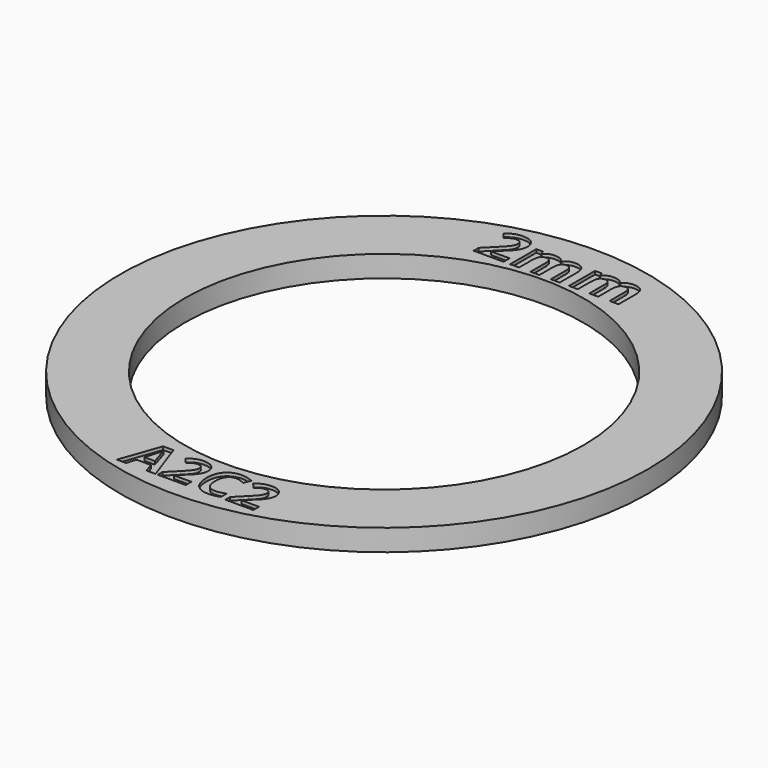
from build123d import *

# Parameters (mm, degrees)
F0_R           = 24.5
F0_R_2         = 18.5
F0_TEXT_SIZE   = 5.1974965673
F0_TEXT_SIZE_2 = 5.5555555556
F1_DEPTH       = 2
F2_DEPTH       = 0.3


# Not quite as in the source:
# - Text() gives the source's letters only with a copy of the font that has no kerning and outlines rounded to 1/6400 em; it was checked with that copy


with BuildPart() as f1:
    # F0 (on Top) → F1 (new body)
    with BuildSketch(Plane.XY):
        Circle(F0_R)
        Polygon((-2.9154707307, -22.8730905801), (-3.7633123583, -22.8730905801), (-4.0321203839, -21.9895161637), (-5.3850937091, -21.9895161637), (-5.6539017347, -22.8730905801), (-6.5017433622, -22.8730905801), (-5.1918118055, -19.1471352284), (-4.2302749405, -19.1471352284), align=None, mode=Mode.SUBTRACT)
        with BuildLine():
            Line((-0.1136952374, -22.2128460943), (-0.1136952374, -22.8730905801))
            Line((-0.1136952374, -22.8730905801), (-2.707570868, -22.8730905801))
            Line((-2.707570868, -22.8730905801), (-2.707570868, -22.3273534405))
            Line((-2.707570868, -22.3273534405), (-1.7760820301, -21.3861192965))
            add(Edge.make_bspline(
                [(-1.7760820301, -21.3861192965), (-1.3619065224, -20.9621984828), (-1.2352175436, -20.7985585518)],
                knots=[0, 0, 0, 1, 1, 1], degree=2))
            add(Edge.make_bspline(
                [(-1.2352175436, -20.7985585518), (-1.1085285648, -20.6349186208), (-1.0524930549, -20.4952359005)],
                knots=[0, 0, 0, 1, 1, 1], degree=2))
            add(Edge.make_bspline(
                [(-1.0524930549, -20.4952359005), (-0.996457545, -20.3555531803), (-0.996457545, -20.206125154)],
                knots=[0, 0, 0, 1, 1, 1], degree=2))
            add(Edge.make_bspline(
                [(-0.996457545, -20.206125154), (-0.996457545, -19.9827952234), (-1.1198980885, -19.8735665846)],
                knots=[0, 0, 0, 1, 1, 1], degree=2))
            add(Edge.make_bspline(
                [(-1.1198980885, -19.8735665846), (-1.243338632, -19.7643379458), (-1.4488021681, -19.7643379458)],
                knots=[0, 0, 0, 1, 1, 1], degree=2))
            add(Edge.make_bspline(
                [(-1.4488021681, -19.7643379458), (-1.6640110104, -19.7643379458), (-1.86703822, -19.8634152241)],
                knots=[0, 0, 0, 1, 1, 1], degree=2))
            add(Edge.make_bspline(
                [(-1.86703822, -19.8634152241), (-2.0700654297, -19.9624925024), (-2.2909590338, -20.1452169911)],
                knots=[0, 0, 0, 1, 1, 1], degree=2))
            Line((-2.2909590338, -20.1452169911), (-2.7173161741, -19.6400852935))
            add(Edge.make_bspline(
                [(-2.7173161741, -19.6400852935), (-2.4436354955, -19.4061979479), (-2.2633473333, -19.3099630505)],
                knots=[0, 0, 0, 1, 1, 1], degree=2))
            add(Edge.make_bspline(
                [(-2.2633473333, -19.3099630505), (-2.0830591711, -19.2137281532), (-1.869880601, -19.1617531875)],
                knots=[0, 0, 0, 1, 1, 1], degree=2))
            add(Edge.make_bspline(
                [(-1.869880601, -19.1617531875), (-1.6567020308, -19.1097782218), (-1.3927666583, -19.1097782218)],
                knots=[0, 0, 0, 1, 1, 1], degree=2))
            add(Edge.make_bspline(
                [(-1.3927666583, -19.1097782218), (-1.0451840753, -19.1097782218), (-0.7788123763, -19.2364672006)],
                knots=[0, 0, 0, 1, 1, 1], degree=2))
            add(Edge.make_bspline(
                [(-0.7788123763, -19.2364672006), (-0.5124406772, -19.3631561795), (-0.365042923, -19.5917648176)],
                knots=[0, 0, 0, 1, 1, 1], degree=2))
            add(Edge.make_bspline(
                [(-0.365042923, -19.5917648176), (-0.2176451688, -19.8203734556), (-0.2176451688, -20.1143568552)],
                knots=[0, 0, 0, 1, 1, 1], degree=2))
            add(Edge.make_bspline(
                [(-0.2176451688, -20.1143568552), (-0.2176451688, -20.3709832482), (-0.3077892498, -20.5955313421)],
                knots=[0, 0, 0, 1, 1, 1], degree=2))
            add(Edge.make_bspline(
                [(-0.3077892498, -20.5955313421), (-0.3979333309, -20.820079436), (-0.5871546903, -21.0559970536)],
                knots=[0, 0, 0, 1, 1, 1], degree=2))
            add(Edge.make_bspline(
                [(-0.5871546903, -21.0559970536), (-0.7763760497, -21.2919146713), (-1.253083938, -21.7288292265)],
                knots=[0, 0, 0, 1, 1, 1], degree=2))
            Line((-1.253083938, -21.7288292265), (-1.7306039352, -22.1779254142))
            Line((-1.7306039352, -22.1779254142), (-1.7306039352, -22.2128460943))
            Line((-1.7306039352, -22.2128460943), (-0.1136952374, -22.2128460943))
        make_face(mode=Mode.SUBTRACT)
        Circle(F0_R_2, mode=Mode.SUBTRACT)
        with BuildLine():
            add(Edge.make_bspline(
                [(2.5077920937, -19.8378337957), (2.2974559045, -19.7643379458), (2.0944286949, -19.7643379458)],
                knots=[0, 0, 0, 1, 1, 1], degree=2))
            add(Edge.make_bspline(
                [(2.0944286949, -19.7643379458), (1.6502051601, -19.7643379458), (1.4065725085, -20.0981146785)],
                knots=[0, 0, 0, 1, 1, 1], degree=2))
            add(Edge.make_bspline(
                [(1.4065725085, -20.0981146785), (1.1629398569, -20.4318914111), (1.1629398569, -21.0279792987)],
                knots=[0, 0, 0, 1, 1, 1], degree=2))
            add(Edge.make_bspline(
                [(1.1629398569, -21.0279792987), (1.1629398569, -22.2688816042), (2.0944286949, -22.2688816042)],
                knots=[0, 0, 0, 1, 1, 1], degree=2))
            add(Edge.make_bspline(
                [(2.0944286949, -22.2688816042), (2.4850530463, -22.2688816042), (3.0405354919, -22.0739754829)],
                knots=[0, 0, 0, 1, 1, 1], degree=2))
            Line((3.0405354919, -22.0739754829), (3.0405354919, -22.7334078599))
            add(Edge.make_bspline(
                [(3.0405354919, -22.7334078599), (2.5841303246, -22.9242534369), (2.0205267906, -22.9242534369)],
                knots=[0, 0, 0, 1, 1, 1], degree=2))
            add(Edge.make_bspline(
                [(2.0205267906, -22.9242534369), (1.2108542784, -22.9242534369), (0.7820608116, -22.4329275896)],
                knots=[0, 0, 0, 1, 1, 1], degree=2))
            add(Edge.make_bspline(
                [(0.7820608116, -22.4329275896), (0.3532673448, -21.9416017422), (0.3532673448, -21.0231066457)],
                knots=[0, 0, 0, 1, 1, 1], degree=2))
            add(Edge.make_bspline(
                [(0.3532673448, -21.0231066457), (0.3532673448, -20.4440730437), (0.5640095884, -20.0087827062)],
                knots=[0, 0, 0, 1, 1, 1], degree=2))
            add(Edge.make_bspline(
                [(0.5640095884, -20.0087827062), (0.7747518321, -19.5734923687), (1.1694367277, -19.3416352953)],
                knots=[0, 0, 0, 1, 1, 1], degree=2))
            add(Edge.make_bspline(
                [(1.1694367277, -19.3416352953), (1.5641216232, -19.1097782218), (2.0944286949, -19.1097782218)],
                knots=[0, 0, 0, 1, 1, 1], degree=2))
            add(Edge.make_bspline(
                [(2.0944286949, -19.1097782218), (2.6344810726, -19.1097782218), (3.1802182121, -19.370465159)],
                knots=[0, 0, 0, 1, 1, 1], degree=2))
            Line((3.1802182121, -19.370465159), (2.9268402545, -20.0104069239))
            add(Edge.make_bspline(
                [(2.9268402545, -20.0104069239), (2.7181282829, -19.9113296456), (2.5077920937, -19.8378337957)],
                knots=[0, 0, 0, 1, 1, 1], degree=2))
        make_face(mode=Mode.SUBTRACT)
        with BuildLine():
            Line((6.1647181942, -22.2128460943), (6.1647181942, -22.8730905801))
            Line((6.1647181942, -22.8730905801), (3.5708425635, -22.8730905801))
            Line((3.5708425635, -22.8730905801), (3.5708425635, -22.3273534405))
            Line((3.5708425635, -22.3273534405), (4.5023314015, -21.3861192965))
            add(Edge.make_bspline(
                [(4.5023314015, -21.3861192965), (4.9165069092, -20.9621984828), (5.043195888, -20.7985585518)],
                knots=[0, 0, 0, 1, 1, 1], degree=2))
            add(Edge.make_bspline(
                [(5.043195888, -20.7985585518), (5.1698848668, -20.6349186208), (5.2259203767, -20.4952359005)],
                knots=[0, 0, 0, 1, 1, 1], degree=2))
            add(Edge.make_bspline(
                [(5.2259203767, -20.4952359005), (5.2819558866, -20.3555531803), (5.2819558866, -20.206125154)],
                knots=[0, 0, 0, 1, 1, 1], degree=2))
            add(Edge.make_bspline(
                [(5.2819558866, -20.206125154), (5.2819558866, -19.9827952234), (5.1585153431, -19.8735665846)],
                knots=[0, 0, 0, 1, 1, 1], degree=2))
            add(Edge.make_bspline(
                [(5.1585153431, -19.8735665846), (5.0350747996, -19.7643379458), (4.8296112634, -19.7643379458)],
                knots=[0, 0, 0, 1, 1, 1], degree=2))
            add(Edge.make_bspline(
                [(4.8296112634, -19.7643379458), (4.6144024212, -19.7643379458), (4.4113752115, -19.8634152241)],
                knots=[0, 0, 0, 1, 1, 1], degree=2))
            add(Edge.make_bspline(
                [(4.4113752115, -19.8634152241), (4.2083480019, -19.9624925024), (3.9874543978, -20.1452169911)],
                knots=[0, 0, 0, 1, 1, 1], degree=2))
            Line((3.9874543978, -20.1452169911), (3.5610972575, -19.6400852935))
            add(Edge.make_bspline(
                [(3.5610972575, -19.6400852935), (3.8347779361, -19.4061979479), (4.0150660983, -19.3099630505)],
                knots=[0, 0, 0, 1, 1, 1], degree=2))
            add(Edge.make_bspline(
                [(4.0150660983, -19.3099630505), (4.1953542604, -19.2137281532), (4.4085328306, -19.1617531875)],
                knots=[0, 0, 0, 1, 1, 1], degree=2))
            add(Edge.make_bspline(
                [(4.4085328306, -19.1617531875), (4.6217114007, -19.1097782218), (4.8856467733, -19.1097782218)],
                knots=[0, 0, 0, 1, 1, 1], degree=2))
            add(Edge.make_bspline(
                [(4.8856467733, -19.1097782218), (5.2332293562, -19.1097782218), (5.4996010553, -19.2364672006)],
                knots=[0, 0, 0, 1, 1, 1], degree=2))
            add(Edge.make_bspline(
                [(5.4996010553, -19.2364672006), (5.7659727544, -19.3631561795), (5.9133705086, -19.5917648176)],
                knots=[0, 0, 0, 1, 1, 1], degree=2))
            add(Edge.make_bspline(
                [(5.9133705086, -19.5917648176), (6.0607682628, -19.8203734556), (6.0607682628, -20.1143568552)],
                knots=[0, 0, 0, 1, 1, 1], degree=2))
            add(Edge.make_bspline(
                [(6.0607682628, -20.1143568552), (6.0607682628, -20.3709832482), (5.9706241817, -20.5955313421)],
                knots=[0, 0, 0, 1, 1, 1], degree=2))
            add(Edge.make_bspline(
                [(5.9706241817, -20.5955313421), (5.8804801006, -20.820079436), (5.6912587412, -21.0559970536)],
                knots=[0, 0, 0, 1, 1, 1], degree=2))
            add(Edge.make_bspline(
                [(5.6912587412, -21.0559970536), (5.5020373818, -21.2919146713), (5.0253294935, -21.7288292265)],
                knots=[0, 0, 0, 1, 1, 1], degree=2))
            Line((5.0253294935, -21.7288292265), (4.5478094964, -22.1779254142))
            Line((4.5478094964, -22.1779254142), (4.5478094964, -22.2128460943))
            Line((4.5478094964, -22.2128460943), (6.1647181942, -22.2128460943))
        make_face(mode=Mode.SUBTRACT)
        with BuildLine():
            Line((-4.0182291667, 19.590204057), (-4.0182291667, 18.8844748903))
            Line((-4.0182291667, 18.8844748903), (-6.7907986111, 18.8844748903))
            Line((-6.7907986111, 18.8844748903), (-6.7907986111, 19.4678082236))
            Line((-6.7907986111, 19.4678082236), (-5.7951388889, 20.4738846125))
            add(Edge.make_bspline(
                [(-5.7951388889, 20.4738846125), (-5.3524305556, 20.9270096125), (-5.2170138889, 21.101922807)],
                knots=[0, 0, 0, 1, 1, 1], degree=2))
            add(Edge.make_bspline(
                [(-5.2170138889, 21.101922807), (-5.0815972222, 21.2768360014), (-5.0217013889, 21.426141557)],
                knots=[0, 0, 0, 1, 1, 1], degree=2))
            add(Edge.make_bspline(
                [(-5.0217013889, 21.426141557), (-4.9618055556, 21.5754471125), (-4.9618055556, 21.7351693348)],
                knots=[0, 0, 0, 1, 1, 1], degree=2))
            add(Edge.make_bspline(
                [(-4.9618055556, 21.7351693348), (-4.9618055556, 21.9738846125), (-5.09375, 22.0906380848)],
                knots=[0, 0, 0, 1, 1, 1], degree=2))
            add(Edge.make_bspline(
                [(-5.09375, 22.0906380848), (-5.2256944444, 22.207391557), (-5.4453125, 22.207391557)],
                knots=[0, 0, 0, 1, 1, 1], degree=2))
            add(Edge.make_bspline(
                [(-5.4453125, 22.207391557), (-5.6753472222, 22.207391557), (-5.8923611111, 22.1014887792)],
                knots=[0, 0, 0, 1, 1, 1], degree=2))
            add(Edge.make_bspline(
                [(-5.8923611111, 22.1014887792), (-6.109375, 21.9955860014), (-6.3454861111, 21.8002735014)],
                knots=[0, 0, 0, 1, 1, 1], degree=2))
            Line((-6.3454861111, 21.8002735014), (-6.8012152778, 22.340204057))
            add(Edge.make_bspline(
                [(-6.8012152778, 22.340204057), (-6.5086805556, 22.590204057), (-6.3159722222, 22.6930686403)],
                knots=[0, 0, 0, 1, 1, 1], degree=2))
            add(Edge.make_bspline(
                [(-6.3159722222, 22.6930686403), (-6.1232638889, 22.7959332236), (-5.8953993056, 22.8514887792)],
                knots=[0, 0, 0, 1, 1, 1], degree=2))
            add(Edge.make_bspline(
                [(-5.8953993056, 22.8514887792), (-5.6675347222, 22.9070443348), (-5.3854166667, 22.9070443348)],
                knots=[0, 0, 0, 1, 1, 1], degree=2))
            add(Edge.make_bspline(
                [(-5.3854166667, 22.9070443348), (-5.0138888889, 22.9070443348), (-4.7291666667, 22.7716276681)],
                knots=[0, 0, 0, 1, 1, 1], degree=2))
            add(Edge.make_bspline(
                [(-4.7291666667, 22.7716276681), (-4.4444444444, 22.6362110014), (-4.2868923611, 22.3918533625)],
                knots=[0, 0, 0, 1, 1, 1], degree=2))
            add(Edge.make_bspline(
                [(-4.2868923611, 22.3918533625), (-4.1293402778, 22.1474957236), (-4.1293402778, 21.8332596125)],
                knots=[0, 0, 0, 1, 1, 1], degree=2))
            add(Edge.make_bspline(
                [(-4.1293402778, 21.8332596125), (-4.1293402778, 21.558954057), (-4.2256944444, 21.3189366959)],
                knots=[0, 0, 0, 1, 1, 1], degree=2))
            add(Edge.make_bspline(
                [(-4.2256944444, 21.3189366959), (-4.3220486111, 21.0789193348), (-4.5243055556, 20.8267491959)],
                knots=[0, 0, 0, 1, 1, 1], degree=2))
            add(Edge.make_bspline(
                [(-4.5243055556, 20.8267491959), (-4.7265625, 20.574579057), (-5.2361111111, 20.1075651681)],
                knots=[0, 0, 0, 1, 1, 1], degree=2))
            Line((-5.2361111111, 20.1075651681), (-5.7465277778, 19.6275304459))
            Line((-5.7465277778, 19.6275304459), (-5.7465277778, 19.590204057))
            Line((-5.7465277778, 19.590204057), (-4.0182291667, 19.590204057))
        make_face(mode=Mode.SUBTRACT)
        with BuildLine():
            Line((-0.6927083333, 20.4061762792), (-0.6927083333, 18.8844748903))
            Line((-0.6927083333, 18.8844748903), (-1.5199652778, 18.8844748903))
            Line((-1.5199652778, 18.8844748903), (-1.5199652778, 20.6561762792))
            add(Edge.make_bspline(
                [(-1.5199652778, 20.6561762792), (-1.5199652778, 20.9843012792), (-1.6297743056, 21.1483637792)],
                knots=[0, 0, 0, 1, 1, 1], degree=2))
            add(Edge.make_bspline(
                [(-1.6297743056, 21.1483637792), (-1.7395833333, 21.3124262792), (-1.9756944444, 21.3124262792)],
                knots=[0, 0, 0, 1, 1, 1], degree=2))
            add(Edge.make_bspline(
                [(-1.9756944444, 21.3124262792), (-2.2934027778, 21.3124262792), (-2.4370659722, 21.0789193348)],
                knots=[0, 0, 0, 1, 1, 1], degree=2))
            add(Edge.make_bspline(
                [(-2.4370659722, 21.0789193348), (-2.5807291667, 20.8454123903), (-2.5807291667, 20.3115582236)],
                knots=[0, 0, 0, 1, 1, 1], degree=2))
            Line((-2.5807291667, 20.3115582236), (-2.5807291667, 18.8844748903))
            Line((-2.5807291667, 18.8844748903), (-3.4079861111, 18.8844748903))
            Line((-3.4079861111, 18.8844748903), (-3.4079861111, 21.9174610014))
            Line((-3.4079861111, 21.9174610014), (-2.7760416667, 21.9174610014))
            Line((-2.7760416667, 21.9174610014), (-2.6649305556, 21.5294401681))
            Line((-2.6649305556, 21.5294401681), (-2.6189236111, 21.5294401681))
            add(Edge.make_bspline(
                [(-2.6189236111, 21.5294401681), (-2.4965277778, 21.738641557), (-2.2660590278, 21.8562630848)],
                knots=[0, 0, 0, 1, 1, 1], degree=2))
            add(Edge.make_bspline(
                [(-2.2660590278, 21.8562630848), (-2.0355902778, 21.9738846125), (-1.7369791667, 21.9738846125)],
                knots=[0, 0, 0, 1, 1, 1], degree=2))
            add(Edge.make_bspline(
                [(-1.7369791667, 21.9738846125), (-1.0564236111, 21.9738846125), (-0.8142361111, 21.5294401681)],
                knots=[0, 0, 0, 1, 1, 1], degree=2))
            Line((-0.8142361111, 21.5294401681), (-0.7413194444, 21.5294401681))
            add(Edge.make_bspline(
                [(-0.7413194444, 21.5294401681), (-0.6189236111, 21.7412457236), (-0.3819444444, 21.8575651681)],
                knots=[0, 0, 0, 1, 1, 1], degree=2))
            add(Edge.make_bspline(
                [(-0.3819444444, 21.8575651681), (-0.1449652778, 21.9738846125), (0.1536458333, 21.9738846125)],
                knots=[0, 0, 0, 1, 1, 1], degree=2))
            add(Edge.make_bspline(
                [(0.1536458333, 21.9738846125), (0.6692708333, 21.9738846125), (0.93359375, 21.7095616959)],
                knots=[0, 0, 0, 1, 1, 1], degree=2))
            add(Edge.make_bspline(
                [(0.93359375, 21.7095616959), (1.1979166667, 21.4452387792), (1.1979166667, 20.8619054459)],
                knots=[0, 0, 0, 1, 1, 1], degree=2))
            Line((1.1979166667, 20.8619054459), (1.1979166667, 18.8844748903))
            Line((1.1979166667, 18.8844748903), (0.3680555556, 18.8844748903))
            Line((0.3680555556, 18.8844748903), (0.3680555556, 20.6561762792))
            add(Edge.make_bspline(
                [(0.3680555556, 20.6561762792), (0.3680555556, 20.9843012792), (0.2582465278, 21.1483637792)],
                knots=[0, 0, 0, 1, 1, 1], degree=2))
            add(Edge.make_bspline(
                [(0.2582465278, 21.1483637792), (0.1484375, 21.3124262792), (-0.0876736111, 21.3124262792)],
                knots=[0, 0, 0, 1, 1, 1], degree=2))
            add(Edge.make_bspline(
                [(-0.0876736111, 21.3124262792), (-0.3914930556, 21.3124262792), (-0.5421006944, 21.0954123903)],
                knots=[0, 0, 0, 1, 1, 1], degree=2))
            add(Edge.make_bspline(
                [(-0.5421006944, 21.0954123903), (-0.6927083333, 20.8783985014), (-0.6927083333, 20.4061762792)],
                knots=[0, 0, 0, 1, 1, 1], degree=2))
        make_face(mode=Mode.SUBTRACT)
        with BuildLine():
            Line((4.7621527778, 20.4061762792), (4.7621527778, 18.8844748903))
            Line((4.7621527778, 18.8844748903), (3.9348958333, 18.8844748903))
            Line((3.9348958333, 18.8844748903), (3.9348958333, 20.6561762792))
            add(Edge.make_bspline(
                [(3.9348958333, 20.6561762792), (3.9348958333, 20.9843012792), (3.8250868056, 21.1483637792)],
                knots=[0, 0, 0, 1, 1, 1], degree=2))
            add(Edge.make_bspline(
                [(3.8250868056, 21.1483637792), (3.7152777778, 21.3124262792), (3.4791666667, 21.3124262792)],
                knots=[0, 0, 0, 1, 1, 1], degree=2))
            add(Edge.make_bspline(
                [(3.4791666667, 21.3124262792), (3.1614583333, 21.3124262792), (3.0177951389, 21.0789193348)],
                knots=[0, 0, 0, 1, 1, 1], degree=2))
            add(Edge.make_bspline(
                [(3.0177951389, 21.0789193348), (2.8741319444, 20.8454123903), (2.8741319444, 20.3115582236)],
                knots=[0, 0, 0, 1, 1, 1], degree=2))
            Line((2.8741319444, 20.3115582236), (2.8741319444, 18.8844748903))
            Line((2.8741319444, 18.8844748903), (2.046875, 18.8844748903))
            Line((2.046875, 18.8844748903), (2.046875, 21.9174610014))
            Line((2.046875, 21.9174610014), (2.6788194444, 21.9174610014))
            Line((2.6788194444, 21.9174610014), (2.7899305556, 21.5294401681))
            Line((2.7899305556, 21.5294401681), (2.8359375, 21.5294401681))
            add(Edge.make_bspline(
                [(2.8359375, 21.5294401681), (2.9583333333, 21.738641557), (3.1888020833, 21.8562630848)],
                knots=[0, 0, 0, 1, 1, 1], degree=2))
            add(Edge.make_bspline(
                [(3.1888020833, 21.8562630848), (3.4192708333, 21.9738846125), (3.7178819444, 21.9738846125)],
                knots=[0, 0, 0, 1, 1, 1], degree=2))
            add(Edge.make_bspline(
                [(3.7178819444, 21.9738846125), (4.3984375, 21.9738846125), (4.640625, 21.5294401681)],
                knots=[0, 0, 0, 1, 1, 1], degree=2))
            Line((4.640625, 21.5294401681), (4.7135416667, 21.5294401681))
            add(Edge.make_bspline(
                [(4.7135416667, 21.5294401681), (4.8359375, 21.7412457236), (5.0729166667, 21.8575651681)],
                knots=[0, 0, 0, 1, 1, 1], degree=2))
            add(Edge.make_bspline(
                [(5.0729166667, 21.8575651681), (5.3098958333, 21.9738846125), (5.6085069444, 21.9738846125)],
                knots=[0, 0, 0, 1, 1, 1], degree=2))
            add(Edge.make_bspline(
                [(5.6085069444, 21.9738846125), (6.1241319444, 21.9738846125), (6.3884548611, 21.7095616959)],
                knots=[0, 0, 0, 1, 1, 1], degree=2))
            add(Edge.make_bspline(
                [(6.3884548611, 21.7095616959), (6.6527777778, 21.4452387792), (6.6527777778, 20.8619054459)],
                knots=[0, 0, 0, 1, 1, 1], degree=2))
            Line((6.6527777778, 20.8619054459), (6.6527777778, 18.8844748903))
            Line((6.6527777778, 18.8844748903), (5.8229166667, 18.8844748903))
            Line((5.8229166667, 18.8844748903), (5.8229166667, 20.6561762792))
            add(Edge.make_bspline(
                [(5.8229166667, 20.6561762792), (5.8229166667, 20.9843012792), (5.7131076389, 21.1483637792)],
                knots=[0, 0, 0, 1, 1, 1], degree=2))
            add(Edge.make_bspline(
                [(5.7131076389, 21.1483637792), (5.6032986111, 21.3124262792), (5.3671875, 21.3124262792)],
                knots=[0, 0, 0, 1, 1, 1], degree=2))
            add(Edge.make_bspline(
                [(5.3671875, 21.3124262792), (5.0633680556, 21.3124262792), (4.9127604167, 21.0954123903)],
                knots=[0, 0, 0, 1, 1, 1], degree=2))
            add(Edge.make_bspline(
                [(4.9127604167, 21.0954123903), (4.7621527778, 20.8783985014), (4.7621527778, 20.4061762792)],
                knots=[0, 0, 0, 1, 1, 1], degree=2))
        make_face(mode=Mode.SUBTRACT)
        with BuildLine():
            Line((-5.1869391524, -21.3300837867), (-4.2205296344, -21.3300837867))
            add(Edge.make_bspline(
                [(-4.2205296344, -21.3300837867), (-4.5932875914, -20.1297869232), (-4.640389904, -19.9722378085)],
                knots=[0, 0, 0, 1, 1, 1], degree=2))
            add(Edge.make_bspline(
                [(-4.640389904, -19.9722378085), (-4.6874922167, -19.8146886938), (-4.7077949376, -19.7237325038)],
                knots=[0, 0, 0, 1, 1, 1], degree=2))
            add(Edge.make_bspline(
                [(-4.7077949376, -19.7237325038), (-4.791442148, -20.0485760393), (-5.1869391524, -21.3300837867)],
                knots=[0, 0, 0, 1, 1, 1], degree=2))
        make_face()
        with Locations((-6.5017433622, -22.8730905801)):
            Text('A2C2', F0_TEXT_SIZE, font='Open Sans', font_style=FontStyle.BOLD, text_align=(TextAlign.LEFT, TextAlign.BOTTOM))
        with Locations((-7.0130208333, 18.8844748903)):
            Text('2mm', F0_TEXT_SIZE_2, font='Open Sans', font_style=FontStyle.BOLD, text_align=(TextAlign.LEFT, TextAlign.BOTTOM))
    extrude(amount=-F1_DEPTH)

    # F0 (on Top) → F2 (cut)
    with BuildSketch(Plane.XY):
        with Locations((-6.5017433622, -22.8730905801)):
            Text('A2C2', F0_TEXT_SIZE, font='Open Sans', font_style=FontStyle.BOLD, text_align=(TextAlign.LEFT, TextAlign.BOTTOM))
        with Locations((-7.0130208333, 18.8844748903)):
            Text('2mm', F0_TEXT_SIZE_2, font='Open Sans', font_style=FontStyle.BOLD, text_align=(TextAlign.LEFT, TextAlign.BOTTOM))
    extrude(amount=-F2_DEPTH, mode=Mode.SUBTRACT)


solid = f1.part
